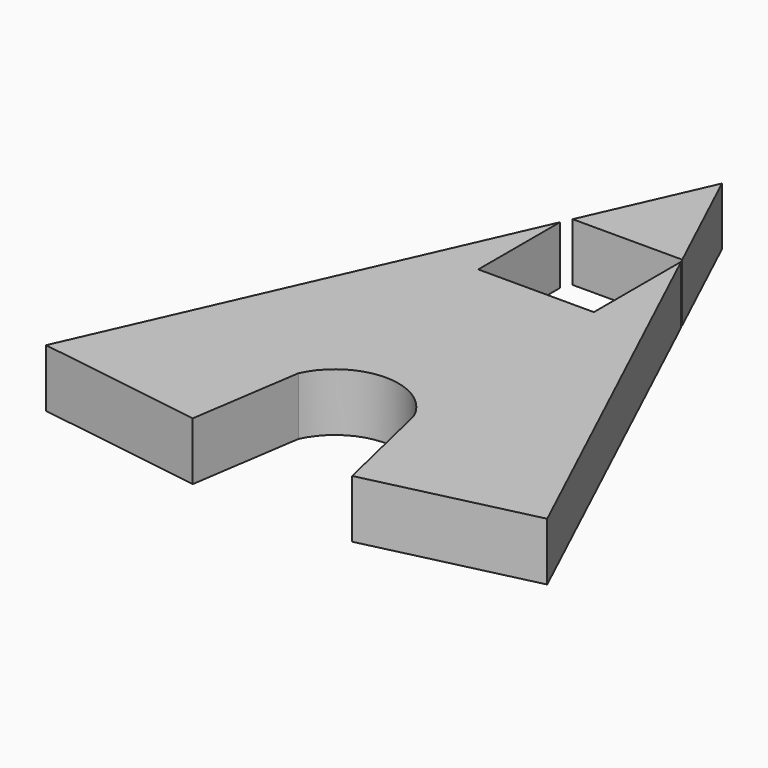
from build123d import *

# Parameters (mm, degrees)
F0_W     = 52.2367432714
F0_H     = 20.7408728629
F1_DEPTH = 26.162


with BuildPart() as f1:
    # F0 (on Top) → F1 (new body)
    with BuildSketch(Plane.XY):
        Polygon((-7.5693419099, -50.2329081684), (0, 0), (0, 30.0591271371), (0, 50.8), (0, 101.6), (0, 147.8053582557), (-82.9187041624, -38.8788953036), align=None)
        Polygon((52.2367432714, 30.0591271371), (52.2367432714, 0), (63.8693667413, -49.4501978884), (138.044663574, -32.0012626835), (52.2367432714, 150.9281977383), (52.2367432714, 101.6), (52.2367432714, 50.8), align=None)
        with BuildLine():
            ThreePointArc((0, 0), (26.1183716357, 16.7427360355), (52.2367432714, 0))
            Line((52.2367432714, 0), (52.2367432714, 30.0591271371))
            Line((52.2367432714, 30.0591271371), (0, 30.0591271371))
            Line((0, 30.0591271371), (0, 0))
        make_face()
        Polygon((0, 50.8), (52.2367432714, 50.8), (26.1183716357, 76.2), align=None)
        Polygon((0, 101.6), (0, 50.8), (26.1183716357, 76.2), align=None)
        Polygon((26.1183716357, 76.2), (52.2367432714, 101.6), (0, 101.6), align=None)
        Polygon((26.1183716357, 76.2), (52.2367432714, 50.8), (52.2367432714, 101.6), align=None)
        with Locations((26.1183716357, 40.4295635685)):
            Rectangle(F0_W, F0_H)
    extrude(amount=F1_DEPTH)


with BuildPart() as f1b:
    # F0 (on Top) → F1, piece 2 (new body)
    with BuildSketch(Plane.XY):
        Polygon((2.0407813314, 152.4), (51.5463553432, 152.4), (26.1183716357, 206.6086012904), align=None)
    extrude(amount=F1_DEPTH)


solid = Compound([f1.part, f1b.part])
